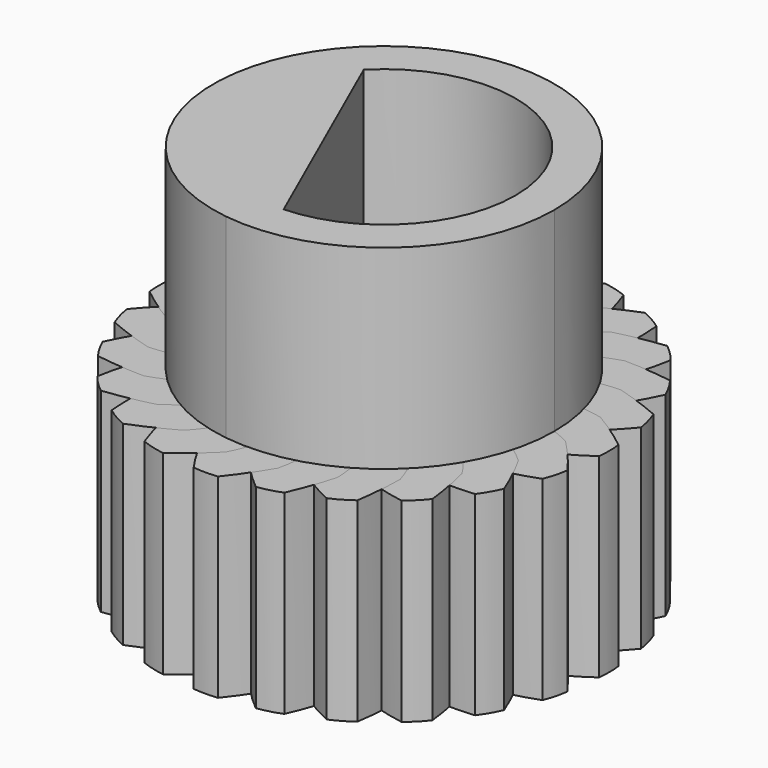
from build123d import *

# Parameters (mm, degrees)
F1_DEPTH = 5
F2_COUNT = 24
F4_DEPTH = 25
F6_DEPTH = 5


# Not quite as in the source:
# - a feature names something its author has since deleted; it is built from what else it names


with BuildPart() as f1:
    # F0 (on Top) → F1 (new body)
    with BuildSketch(Plane.XY):
        with BuildLine():
            ThreePointArc((-1.1496291526, 3.9615625467), (-2.4772368423, -3.2983211831), (4.125, 0))
            ThreePointArc((4.125, 0), (3.2472721782, 2.5437862333), (0.9876189573, 4.0050260667))
            ThreePointArc((0.9876189573, 4.0050260667), (0.2022085053, 4.1200408639), (-0.5906898391, 4.0824882748))
            ThreePointArc((-0.5906898391, 4.0824882748), (-0.8722575916, 4.0317231668), (-1.1496291526, 3.9615625467))
        make_face()
        with BuildLine():
            ThreePointArc((-0.5906898391, 4.0824882748), (0.2022085053, 4.1200408639), (0.9876189573, 4.0050260667))
            ThreePointArc((0.9876189573, 4.0050260667), (0.9502713539, 4.3642035188), (0.881710295, 4.7187492377))
            ThreePointArc((0.881710295, 4.7187492377), (0.6085217759, 5.2469351117), (0.2873408002, 5.7473899701))
            ThreePointArc((0.2873408002, 5.7473899701), (-0.0251888294, 5.7658418103), (-0.3376888711, 5.7468954741))
            ThreePointArc((-0.3376888711, 5.7468954741), (-0.7107512461, 5.2434109952), (-1.0478321475, 4.7151604655))
            ThreePointArc((-1.0478321475, 4.7151604655), (-1.1160740729, 4.3407042786), (-1.1496291526, 3.9615625467))
            ThreePointArc((-1.1496291526, 3.9615625467), (-0.8722575916, 4.0317231668), (-0.5906898391, 4.0824882748))
        make_face()
    extrude(amount=F1_DEPTH)


with BuildPart() as f2_1:
    # F2: instance of F1
    add(f1.part.rotate(Axis((0, 0, 0), (0, 0, -1)), 1 * 360 / F2_COUNT))


with BuildPart() as f2_2:
    # F2: instance of F1
    add(f1.part.rotate(Axis((0, 0, 0), (0, 0, -1)), 2 * 360 / F2_COUNT))


with BuildPart() as f2_3:
    # F2: instance of F1
    add(f1.part.rotate(Axis((0, 0, 0), (0, 0, -1)), 3 * 360 / F2_COUNT))


with BuildPart() as f2_4:
    # F2: instance of F1
    add(f1.part.rotate(Axis((0, 0, 0), (0, 0, -1)), 4 * 360 / F2_COUNT))


with BuildPart() as f2_5:
    # F2: instance of F1
    add(f1.part.rotate(Axis((0, 0, 0), (0, 0, -1)), 5 * 360 / F2_COUNT))


with BuildPart() as f2_6:
    # F2: instance of F1
    add(f1.part.rotate(Axis((0, 0, 0), (0, 0, -1)), 6 * 360 / F2_COUNT))


with BuildPart() as f2_7:
    # F2: instance of F1
    add(f1.part.rotate(Axis((0, 0, 0), (0, 0, -1)), 7 * 360 / F2_COUNT))


with BuildPart() as f2_8:
    # F2: instance of F1
    add(f1.part.rotate(Axis((0, 0, 0), (0, 0, -1)), 8 * 360 / F2_COUNT))


with BuildPart() as f2_9:
    # F2: instance of F1
    add(f1.part.rotate(Axis((0, 0, 0), (0, 0, -1)), 9 * 360 / F2_COUNT))


with BuildPart() as f2_10:
    # F2: instance of F1
    add(f1.part.rotate(Axis((0, 0, 0), (0, 0, -1)), 10 * 360 / F2_COUNT))


with BuildPart() as f2_11:
    # F2: instance of F1
    add(f1.part.rotate(Axis((0, 0, 0), (0, 0, -1)), 11 * 360 / F2_COUNT))


with BuildPart() as f2_12:
    # F2: instance of F1
    add(f1.part.rotate(Axis((0, 0, 0), (0, 0, -1)), 12 * 360 / F2_COUNT))


with BuildPart() as f2_13:
    # F2: instance of F1
    add(f1.part.rotate(Axis((0, 0, 0), (0, 0, -1)), 13 * 360 / F2_COUNT))


with BuildPart() as f2_14:
    # F2: instance of F1
    add(f1.part.rotate(Axis((0, 0, 0), (0, 0, -1)), 14 * 360 / F2_COUNT))


with BuildPart() as f2_15:
    # F2: instance of F1
    add(f1.part.rotate(Axis((0, 0, 0), (0, 0, -1)), 15 * 360 / F2_COUNT))


with BuildPart() as f2_16:
    # F2: instance of F1
    add(f1.part.rotate(Axis((0, 0, 0), (0, 0, -1)), 16 * 360 / F2_COUNT))


with BuildPart() as f2_17:
    # F2: instance of F1
    add(f1.part.rotate(Axis((0, 0, 0), (0, 0, -1)), 17 * 360 / F2_COUNT))


with BuildPart() as f2_18:
    # F2: instance of F1
    add(f1.part.rotate(Axis((0, 0, 0), (0, 0, -1)), 18 * 360 / F2_COUNT))


with BuildPart() as f2_19:
    # F2: instance of F1
    add(f1.part.rotate(Axis((0, 0, 0), (0, 0, -1)), 19 * 360 / F2_COUNT))


with BuildPart() as f2_20:
    # F2: instance of F1
    add(f1.part.rotate(Axis((0, 0, 0), (0, 0, -1)), 20 * 360 / F2_COUNT))


with BuildPart() as f2_21:
    # F2: instance of F1
    add(f1.part.rotate(Axis((0, 0, 0), (0, 0, -1)), 21 * 360 / F2_COUNT))


with BuildPart() as f2_22:
    # F2: instance of F1
    add(f1.part.rotate(Axis((0, 0, 0), (0, 0, -1)), 22 * 360 / F2_COUNT))


with BuildPart() as f2_23:
    # F2: instance of F1
    add(f1.part.rotate(Axis((0, 0, 0), (0, 0, -1)), 23 * 360 / F2_COUNT))


with BuildPart() as f4_tool:
    # F3 (on face) → F4 (new body)
    with BuildSketch(Plane.XY.offset(5)):
        with BuildLine():
            ThreePointArc((0, 3.375), (-1.3070205116, 3.1116430358), (-2.4100629763, 2.3626725229))
            Line((-2.4100629763, 2.3626725229), (0.1230840147, -3.372754857))
            ThreePointArc((0.1230840147, -3.372754857), (2.4296124742, -2.3425644549), (3.375, 0))
            ThreePointArc((3.375, 0), (2.3864853865, 2.3864853865), (0, 3.375))
        make_face()
    extrude(amount=-F4_DEPTH)


with BuildPart() as f1_1:
    add(f1.part)

    # F4: cut by f4_tool
    add(f4_tool.part, mode=Mode.SUBTRACT)


with BuildPart() as f2_1_1:
    add(f2_1.part)

    # F4: cut by f4_tool
    add(f4_tool.part, mode=Mode.SUBTRACT)


with BuildPart() as f2_2_1:
    add(f2_2.part)

    # F4: cut by f4_tool
    add(f4_tool.part, mode=Mode.SUBTRACT)


with BuildPart() as f2_3_1:
    add(f2_3.part)

    # F4: cut by f4_tool
    add(f4_tool.part, mode=Mode.SUBTRACT)


with BuildPart() as f2_4_1:
    add(f2_4.part)

    # F4: cut by f4_tool
    add(f4_tool.part, mode=Mode.SUBTRACT)


with BuildPart() as f2_5_1:
    add(f2_5.part)

    # F4: cut by f4_tool
    add(f4_tool.part, mode=Mode.SUBTRACT)


with BuildPart() as f2_6_1:
    add(f2_6.part)

    # F4: cut by f4_tool
    add(f4_tool.part, mode=Mode.SUBTRACT)


with BuildPart() as f2_7_1:
    add(f2_7.part)

    # F4: cut by f4_tool
    add(f4_tool.part, mode=Mode.SUBTRACT)


with BuildPart() as f2_8_1:
    add(f2_8.part)

    # F4: cut by f4_tool
    add(f4_tool.part, mode=Mode.SUBTRACT)


with BuildPart() as f2_9_1:
    add(f2_9.part)

    # F4: cut by f4_tool
    add(f4_tool.part, mode=Mode.SUBTRACT)


with BuildPart() as f2_10_1:
    add(f2_10.part)

    # F4: cut by f4_tool
    add(f4_tool.part, mode=Mode.SUBTRACT)


with BuildPart() as f2_11_1:
    add(f2_11.part)

    # F4: cut by f4_tool
    add(f4_tool.part, mode=Mode.SUBTRACT)


with BuildPart() as f2_12_1:
    add(f2_12.part)

    # F4: cut by f4_tool
    add(f4_tool.part, mode=Mode.SUBTRACT)


with BuildPart() as f2_13_1:
    add(f2_13.part)

    # F4: cut by f4_tool
    add(f4_tool.part, mode=Mode.SUBTRACT)


with BuildPart() as f2_14_1:
    add(f2_14.part)

    # F4: cut by f4_tool
    add(f4_tool.part, mode=Mode.SUBTRACT)


with BuildPart() as f2_15_1:
    add(f2_15.part)

    # F4: cut by f4_tool
    add(f4_tool.part, mode=Mode.SUBTRACT)


with BuildPart() as f2_16_1:
    add(f2_16.part)

    # F4: cut by f4_tool
    add(f4_tool.part, mode=Mode.SUBTRACT)


with BuildPart() as f2_17_1:
    add(f2_17.part)

    # F4: cut by f4_tool
    add(f4_tool.part, mode=Mode.SUBTRACT)


with BuildPart() as f2_18_1:
    add(f2_18.part)

    # F4: cut by f4_tool
    add(f4_tool.part, mode=Mode.SUBTRACT)


with BuildPart() as f2_19_1:
    add(f2_19.part)

    # F4: cut by f4_tool
    add(f4_tool.part, mode=Mode.SUBTRACT)


with BuildPart() as f2_20_1:
    add(f2_20.part)

    # F4: cut by f4_tool
    add(f4_tool.part, mode=Mode.SUBTRACT)


with BuildPart() as f2_21_1:
    add(f2_21.part)

    # F4: cut by f4_tool
    add(f4_tool.part, mode=Mode.SUBTRACT)


with BuildPart() as f2_22_1:
    add(f2_22.part)

    # F4: cut by f4_tool
    add(f4_tool.part, mode=Mode.SUBTRACT)


with BuildPart() as f2_23_1:
    add(f2_23.part)

    # F4: cut by f4_tool
    add(f4_tool.part, mode=Mode.SUBTRACT)


with BuildPart() as f6:
    # F5 (on face) → F6 (new body)
    with BuildSketch(Plane.XY.offset(5)):
        with BuildLine():
            ThreePointArc((-3.1564365679, 1.1947942051), (0.6073102927, 3.3199095181), (3.375, 0))
            ThreePointArc((3.375, 0), (1.9489484965, -2.7553992012), (-1.1240961529, -3.1822999292))
            Line((-1.1240961529, -3.1822999292), (-0.5887904436, -4.3351990512))
            ThreePointArc((-0.5887904436, -4.3351990512), (2.8779043425, -3.295192194), (4.375, 0))
            ThreePointArc((4.375, 0), (1.2225490863, 4.200714074), (-3.6917422773, 2.3476933271))
            Line((-3.6917422773, 2.3476933271), (-3.1564365679, 1.1947942051))
        make_face()
        with BuildLine():
            ThreePointArc((-1.1240961529, -3.1822999292), (-3.0611237085, -1.4213186277), (-3.1564365679, 1.1947942051))
            Line((-3.1564365679, 1.1947942051), (-3.6917422773, 2.3476933271))
            ThreePointArc((-3.6917422773, 2.3476933271), (-3.9681233258, -1.842450073), (-0.5887904436, -4.3351990512))
            Line((-0.5887904436, -4.3351990512), (-1.1240961529, -3.1822999292))
        make_face()
        with BuildLine():
            Line((0.1230840147, -3.372754857), (-2.4100629763, 2.3626725229))
            ThreePointArc((-2.4100629763, 2.3626725229), (-2.843846732, 1.8174599761), (-3.1564365679, 1.1947942051))
            Line((-3.1564365679, 1.1947942051), (-1.1240961529, -3.1822999292))
            ThreePointArc((-1.1240961529, -3.1822999292), (-0.5094846367, -3.3363228868), (0.1230840147, -3.372754857))
        make_face()
        with BuildLine():
            Line((-1.1240961529, -3.1822999292), (-3.1564365679, 1.1947942051))
            ThreePointArc((-3.1564365679, 1.1947942051), (-3.0611237085, -1.4213186277), (-1.1240961529, -3.1822999292))
        make_face()
    extrude(amount=F6_DEPTH)


solid = Compound([f1_1.part, f2_1_1.part, f2_2_1.part, f2_3_1.part, f2_4_1.part, f2_5_1.part, f2_6_1.part, f2_7_1.part, f2_8_1.part, f2_9_1.part, f2_10_1.part, f2_11_1.part, f2_12_1.part, f2_13_1.part, f2_14_1.part, f2_15_1.part, f2_16_1.part, f2_17_1.part, f2_18_1.part, f2_19_1.part, f2_20_1.part, f2_21_1.part, f2_22_1.part, f2_23_1.part, f6.part])
